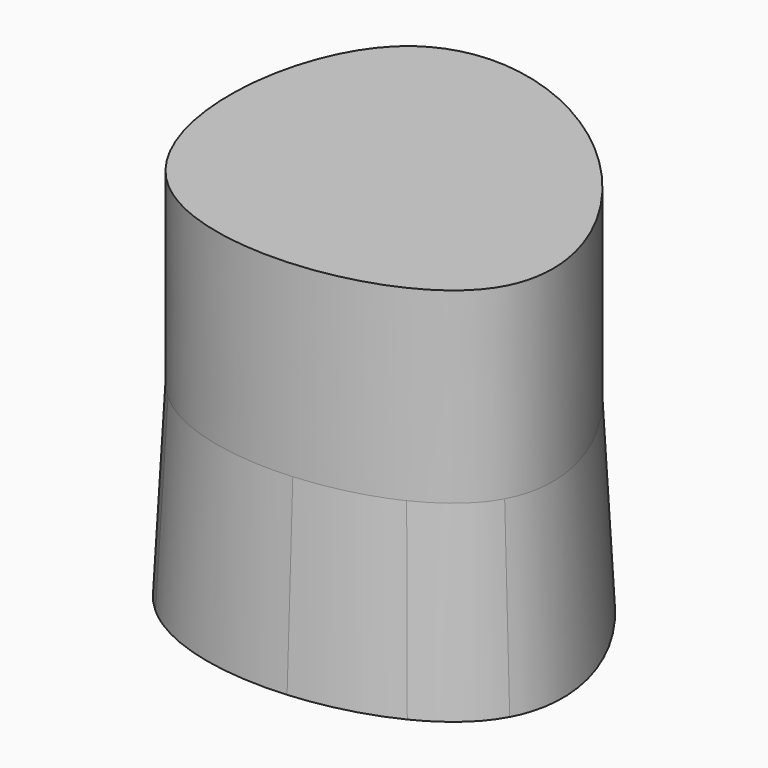
from build123d import *

# Parameters (mm, degrees)
F1_DEPTH = 25
F2_DEPTH = 25
F2_TAPER = -3


with BuildPart() as f1:
    # F0 (on Top) → F1 (new body)
    with BuildSketch(Plane.XY):
        with BuildLine():
            add(Edge.make_bspline(
                [(-4.6990965493, 13.5734938085), (-12.9152492102, 5.4214548467), (-15.5310429084, -38.0420279336), (52.1204516347, -29.5256190924), (28.4129660713, 14.362196757), (2.4999675643, 20.7163809438), (-4.6990965493, 13.5734938085)],
                knots=[0, 0, 0, 0, 0.2604097414, 0.5275806089, 0.7718267294, 1, 1, 1, 1], degree=3))
        make_face()
    extrude(amount=F1_DEPTH)

    # F1_face (on face) → F2 (join)
    with BuildSketch(Plane(origin=(12.860294398, -8.1128243439, 0), x_dir=(1, 0, 0), z_dir=(0, 0, -1))):
        with BuildLine():
            add(Edge.make_bspline(
                [(-17.5593909473, -21.6863181524), (-25.7755436082, -13.5342791906), (-28.3913373064, 29.9292035897), (39.2601572368, 21.4127947484), (15.5526716733, -22.475021101), (-10.3603268337, -28.8292052877), (-17.5593909473, -21.6863181524)],
                knots=[0, 0, 0, 0, 0.2604097414, 0.5275806089, 0.7718267294, 1, 1, 1, 1], degree=3))
        make_face()
    extrude(amount=F2_DEPTH, taper=F2_TAPER)


solid = f1.part
